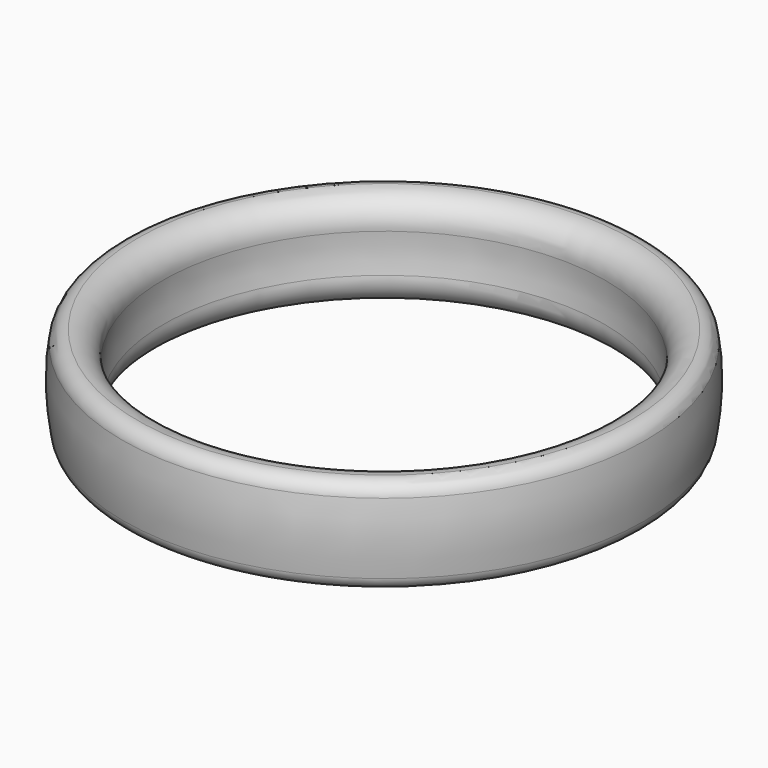
from build123d import *


# Not quite as in the source:
# - a feature names something its author has since deleted; it is built from what else it names


with BuildPart() as f2:
    # F1 (on Front) → F2 (revolve)
    with BuildSketch(Plane.XZ):
        with BuildLine():
            add(Edge.make_bspline(
                [(26.1263029407, 3.5758643896), (26.5604794287, 1.1401700187), (26.3847344036, -1.2152037465), (26.0251071477, -3.5412733739)],
                knots=[1.218218385, 1.218218385, 1.218218385, 1.218218385, 8.3437574948, 8.3437574948, 8.3437574948, 8.3437574948], degree=3))
            ThreePointArc((26.1263029407, 3.5758643896), (25.604469755, 4.4767856269), (24.6259534188, 4.8324184843))
            ThreePointArc((24.6259534188, 4.8324184843), (22.7141751468, 3.9647533307), (22.1085255267, 1.9545474911))
            add(Edge.make_bspline(
                [(22.1085255267, 1.9545474911), (22.2776988691, 0.6940613902), (22.2244853035, -0.6154217727), (22.0138910514, -1.8728684042)],
                knots=[2.940850894, 2.940850894, 2.940850894, 2.940850894, 6.6189607965, 6.6189607965, 6.6189607965, 6.6189607965], degree=3))
            ThreePointArc((22.0138910514, -1.8728684042), (22.580283086, -3.9334460277), (24.5190013744, -4.8324184843))
            ThreePointArc((24.5190013744, -4.8324184843), (25.5108948032, -4.4654506471), (26.0251071477, -3.5412733739))
        make_face()
    revolve(axis=Axis((0, 0, -3.2098824158), (0, 0, -1)))


solid = f2.part
